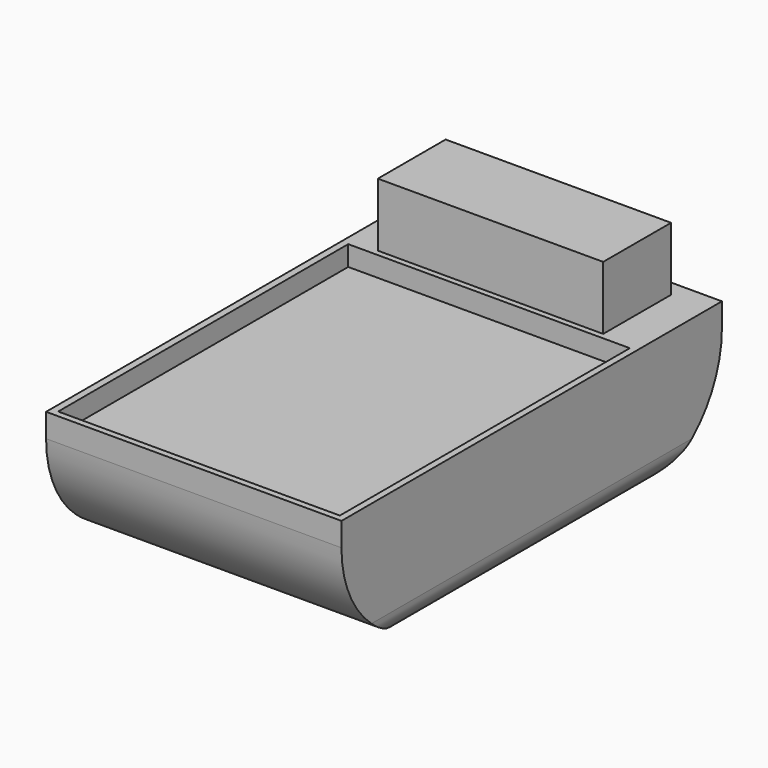
from build123d import *

# Parameters (mm, degrees)
F0_W        = 55.9
F0_H        = 90
F1_DEPTH    = 25
F2_R        = 20.5208152802
F3_W        = 53.3
F3_H        = 68.6
F4_DEPTH    = 3.8
F5_T1_DEPTH = 91.4583694397
F6_T1_DEPTH = 91.4583694397
F8_DEPTH    = 12


# Not quite as in the source:
# - a fillet or chamfer that OpenCascade refuses, or shapes differently, is made with other operations: its cross-section is extruded or revolved along the edge and cut away or added


with BuildPart() as f1:
    # F0 (on Top) → F1 (new body)
    with BuildSketch(Plane.XY):
        with Locations((2.1647780098, -0.8441807004)):
            Rectangle(F0_W, F0_H)
    extrude(amount=F1_DEPTH)

    # F2
    f2_edges = [f1.edges().sort_by_distance(p)[0] for p in [
        (2.164778, -45.844181, 0),
        (2.164778, 44.155819, 0),
    ]]
    fillet(f2_edges, radius=F2_R)

    # F3 (on face) → F4 (cut)
    with BuildSketch(Plane.XY.offset(25)):
        with Locations((2.2094916642, -10.3566651821)):
            Rectangle(F3_W, F3_H)
    extrude(amount=-F4_DEPTH, mode=Mode.SUBTRACT)

    # F5: fillet of radius 5 on 1 edges, made by hand

    # F5_s2 → F5_t1 (cut)
    with BuildSketch(Plane.XZ.offset(-44.8850040195)):
        with BuildLine():
            ThreePointArc((25.1147780098, 0), (28.6503119157, 1.4644660941), (30.1147780098, 5))
            Line((30.1147780098, 5), (30.1147780098, 0))
            Line((30.1147780098, 0), (25.1147780098, 0))
        make_face()
    extrude(amount=F5_T1_DEPTH, mode=Mode.SUBTRACT)

    # F6: fillet of radius 5 on 1 edges, made by hand

    # F6_s2 → F6_t1 (cut)
    with BuildSketch(Plane.XZ.offset(-44.8850040195)):
        with BuildLine():
            ThreePointArc((-25.7852219902, 5), (-24.3207558961, 1.4644660941), (-20.7852219902, 0))
            Line((-20.7852219902, 0), (-25.7852219902, 0))
            Line((-25.7852219902, 0), (-25.7852219902, 5))
        make_face()
    extrude(amount=F6_T1_DEPTH, mode=Mode.SUBTRACT)

    # F7 (on face) → F8 (join)
    with BuildSketch(Plane.XY.offset(25)):
        Polygon((22.9460150003, 41.0868413746), (-19.7153221816, 41.0868413746), (-19.7153221816, 25.0466242433), (22.930214506, 25.0466242433), align=None)
    extrude(amount=F8_DEPTH)


solid = f1.part
